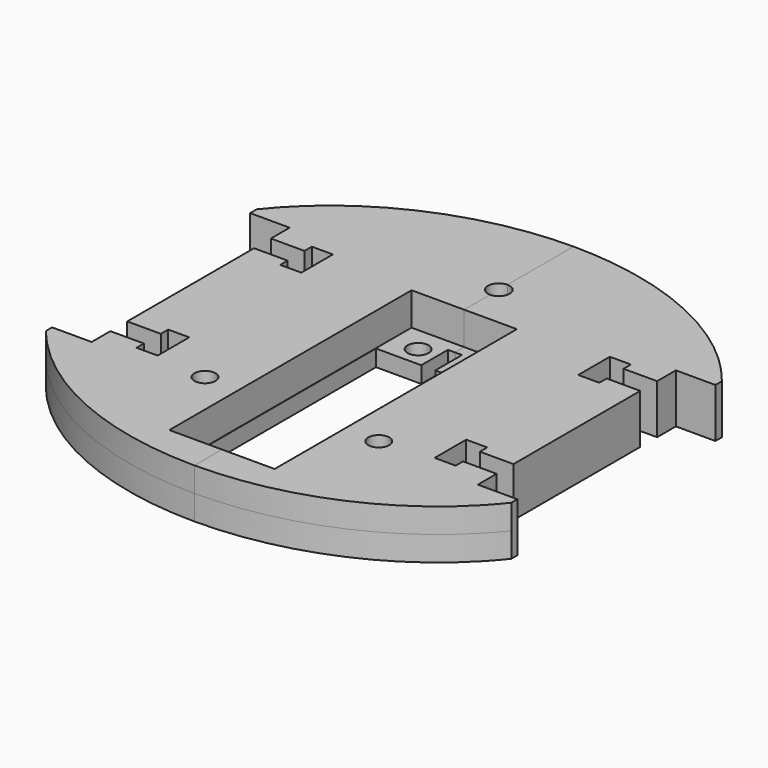
from build123d import *
from build123d import SkipClean  # not in build123d's __all__

# Parameters (mm, degrees)
F0_R     = 2.032
F1_DEPTH = 4.7625
F2_W     = 10.16
F2_H     = 58.42
F3_DEPTH = 6.35


with BuildPart() as f1:
    # F0 (on Top) → F1 (new body, symmetric)
    with BuildSketch(Plane.XY):
        with BuildLine():
            Line((0, -37.2616276145), (0, -45.72))
            add(Edge.make_bspline(
                [(0, -45.72), (28.8508510644, -45.72), (44.8791016558, -25.4)],
                knots=[1.5707963268, 1.5707963268, 1.5707963268, 2.5525616834, 2.5525616834, 2.5525616834], degree=2, weights=[1, 0.8819171037, 1]))
            Line((44.8791016558, -25.4), (44.8791016558, -23.9395))
            Line((44.8791016558, -23.9395), (37.2591016558, -23.9395))
            Line((37.2591016558, -23.9395), (37.2591016558, -19.4183))
            Line((37.2591016558, -19.4183), (30.7821016558, -19.4183))
            Line((30.7821016558, -19.4183), (30.7821016558, -21.1963))
            Line((30.7821016558, -21.1963), (26.7181016558, -21.1963))
            Line((26.7181016558, -21.1963), (26.7181016558, -13.5763))
            Line((26.7181016558, -13.5763), (30.7821016558, -13.5763))
            Line((30.7821016558, -13.5763), (30.7821016558, -15.3543))
            Line((30.7821016558, -15.3543), (37.2591016558, -15.3543))
            Line((37.2591016558, -15.3543), (37.2591016558, 15.2273))
            Line((37.2591016558, 15.2273), (30.7821016558, 15.2273))
            Line((30.7821016558, 15.2273), (30.7821016558, 13.4493))
            Line((30.7821016558, 13.4493), (26.7181016558, 13.4493))
            Line((26.7181016558, 13.4493), (26.7181016558, 21.0693))
            Line((26.7181016558, 21.0693), (30.7821016558, 21.0693))
            Line((30.7821016558, 21.0693), (30.7821016558, 19.2913))
            Line((30.7821016558, 19.2913), (37.2591016558, 19.2913))
            Line((37.2591016558, 19.2913), (37.2591016558, 23.8125))
            Line((37.2591016558, 23.8125), (44.8791016558, 23.8125))
            Line((44.8791016558, 23.8125), (44.8791016558, 25.4))
            add(Edge.make_bspline(
                [(44.8791016558, 25.4), (28.8508510644, 45.72), (0, 45.72)],
                knots=[3.7306236238, 3.7306236238, 3.7306236238, 4.7123889804, 4.7123889804, 4.7123889804], degree=2, weights=[1, 0.8819171037, 1]))
            Line((0, 45.72), (0, 29.7815))
            ThreePointArc((0, 29.7815), (2.0955, 27.686), (0, 25.5905))
            Line((0, 25.5905), (0, 17.1200428158))
            Line((0, 17.1200428158), (1.3565140544, 17.1200428158))
            Line((1.3565140544, 17.1200428158), (1.3565140544, 10.6807))
            Line((1.3565140544, 10.6807), (10.0905383006, 10.6807))
            Line((10.0905383006, 10.6807), (10.0905383006, -29.9593))
            Line((10.0905383006, -29.9593), (1.3565140544, -29.9593))
            Line((1.3565140544, -29.9593), (1.3565140544, -37.2616276145))
            Line((1.3565140544, -37.2616276145), (0, -37.2616276145))
        make_face()
        with Locations((5.0038, -33.7566)):
            Circle(F0_R, mode=Mode.SUBTRACT)
        with Locations((16.764, -22.225)):
            Circle(F0_R, mode=Mode.SUBTRACT)
        with Locations((5.0038, 14.478)):
            Circle(F0_R, mode=Mode.SUBTRACT)
    extrude(amount=F1_DEPTH, both=True)

    # F2 (on face) → F3 (cut)
    with BuildSketch(Plane.XY.offset(4.7625)):
        with Locations((5.08, -9.8651262736)):
            Rectangle(F2_W, F2_H)
    extrude(amount=-F3_DEPTH, mode=Mode.SUBTRACT)

    # F4: F1 across plane


with BuildPart() as f1_1:
    add(f1.part, clean=False)
    with SkipClean():  # cleaning this boolean's faces spoils the solid; the shape is the same uncleaned
        add(f1.part.mirror(Plane.YZ), clean=False)


solid = f1_1.part
